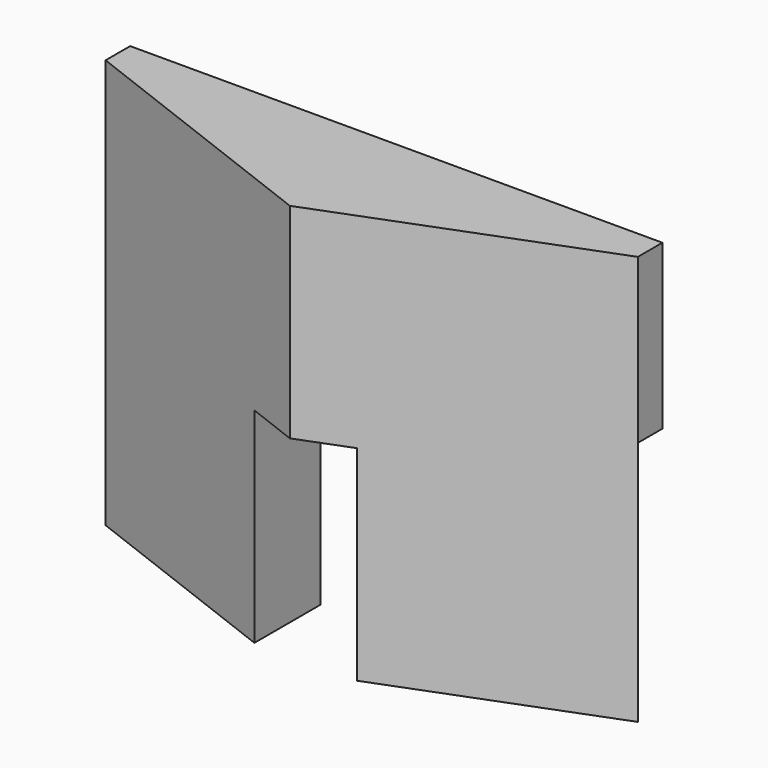
from build123d import *

# Parameters (mm, degrees)
F1_DEPTH = 50.8
F2_W     = 12.7
F2_H     = 25.4
F3_DEPTH = 25.4
F4_W     = 66.04
F4_H     = 20.32
F5_DEPTH = 3.81


# Not quite as in the source:
# - a feature names something its author has since deleted; it is built from what else it names


with BuildPart() as f1:
    # F0 (on Top) → F1 (new body)
    with BuildSketch(Plane.XY):
        Polygon((-3.3912816751, -25.752466172), (-69.4312816751, -25.752466172), (-36.4112816751, -38.452466172), align=None)
    extrude(amount=F1_DEPTH)

    # F2 (on face) → F3 (cut)
    with BuildSketch(Plane(origin=(0, -25.752466172, 0), x_dir=(-1, 0, 0), z_dir=(0, 1, 0))):
        with Locations((36.4112816751, 12.7)):
            Rectangle(F2_W, F2_H)
    extrude(amount=-F3_DEPTH, mode=Mode.SUBTRACT)

    # F4 (on face) → F5 (join)
    with BuildSketch(Plane(origin=(0, -25.752466172, 0), x_dir=(-1, 0, 0), z_dir=(0, 1, 0))):
        with Locations((36.4112816751, 40.64)):
            Rectangle(F4_W, F4_H)
    extrude(amount=F5_DEPTH)


solid = f1.part
